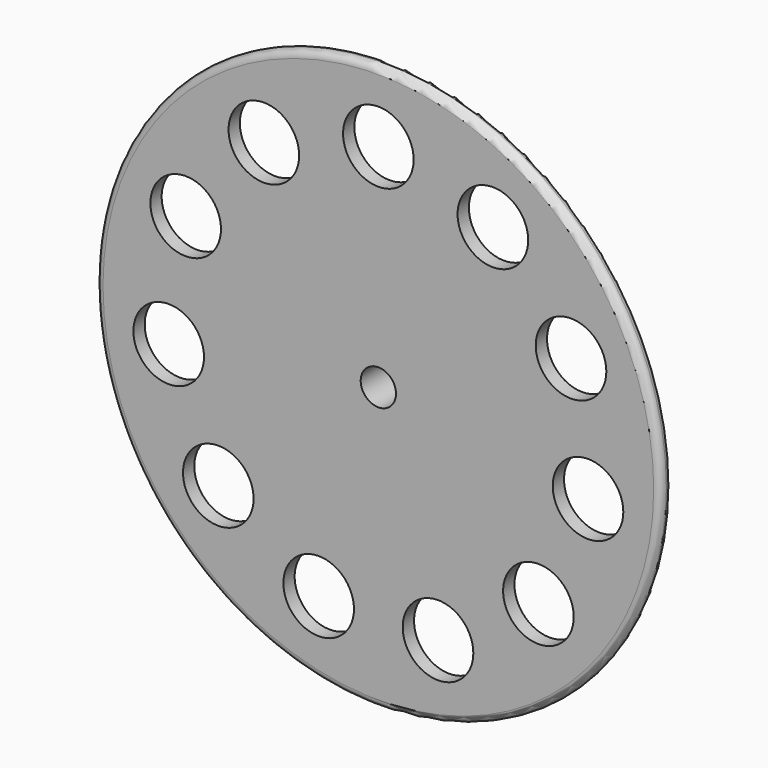
from build123d import *

# Parameters (mm, degrees)
F0_R     = 40
F0_R_2   = 5.0000025111
F0_R_3   = 2.5
F1_DEPTH = 2
F2_R     = 5
F2_R_2   = 2.5
F3_DEPTH = 5
F4_R     = 2.49999
F5_R     = 0.99999


# Not quite as in the source:
# - a fillet or chamfer is up to 0.001 mm smaller than in the source, because OpenCascade refuses the exact size


with BuildPart() as f1:
    # F0 (on Front) → F1 (new body)
    with BuildSketch(Plane.XZ):
        Circle(F0_R)
        with Locations((-8.4519767052, -28.7847892084)):
            Circle(F0_R_2, mode=Mode.SUBTRACT)
        with Locations((-22.6724872306, -19.6458220184)):
            Circle(F0_R_2, mode=Mode.SUBTRACT)
        with Locations((-29.6946432564, -4.2694451482)):
            Circle(F0_R_2, mode=Mode.SUBTRACT)
        with Locations((8.4519767052, -28.7847892084)):
            Circle(F0_R_2, mode=Mode.SUBTRACT)
        with Locations((22.6724872306, -19.6458220184)):
            Circle(F0_R_2, mode=Mode.SUBTRACT)
        with Locations((29.6946432564, -4.2694451482)):
            Circle(F0_R_2, mode=Mode.SUBTRACT)
        with Locations((-27.2889598606, 12.4624503901)):
            Circle(F0_R_2, mode=Mode.SUBTRACT)
        with Locations((-16.2192245237, 25.2376059849)):
            Circle(F0_R_2, mode=Mode.SUBTRACT)
        Circle(F0_R_3, mode=Mode.SUBTRACT)
        with Locations((27.2889598606, 12.4624503901)):
            Circle(F0_R_2, mode=Mode.SUBTRACT)
        with Locations((16.2192245237, 25.2376059849)):
            Circle(F0_R_2, mode=Mode.SUBTRACT)
        with Locations((0, 30)):
            Circle(F0_R_2, mode=Mode.SUBTRACT)
    extrude(amount=F1_DEPTH)

    # F2 (on Front) → F3 (join)
    with BuildSketch(Plane.XZ):
        Circle(F2_R)
        Circle(F2_R_2, mode=Mode.SUBTRACT)
    extrude(amount=-F3_DEPTH)

    # F4 (radius 2.5 in the source; OpenCascade refuses exactly that, so slightly less here)
    f4_edges = [f1.edges().sort_by_distance(p)[0] for p in [
        (-5, 0, 0),
        (-5, 5, 0),
    ]]
    fillet(f4_edges, radius=F4_R)

    # F5 (radius 1 in the source; OpenCascade refuses exactly that, so slightly less here)
    f5_edges = [f1.edges().sort_by_distance(p)[0] for p in [
        (40, -1, 0),
        (-40, 0, 0),
        (-40, -2, 0),
    ]]
    fillet(f5_edges, radius=F5_R)


solid = f1.part
